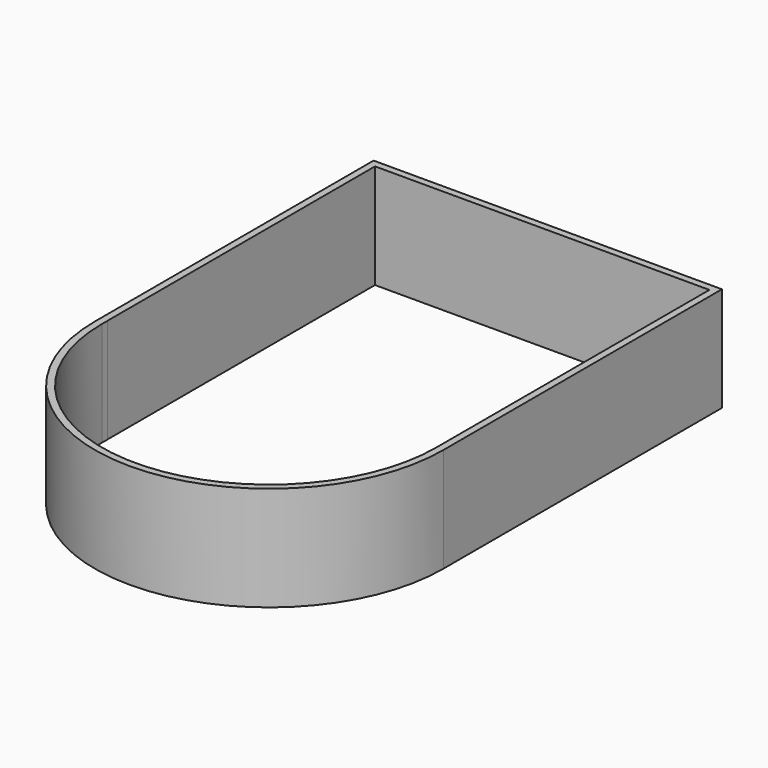
from build123d import *

# Parameters (mm, degrees)
F1_DEPTH = 3000


with BuildPart() as f1:
    # F0 (on Top) → F1 (new body)
    with BuildSketch(Plane.XY):
        with BuildLine():
            Line((5000, 5000), (-5000, 5000))
            Line((-5000, 5000), (-5000, -5000))
            ThreePointArc((-5000, -5000), (-4949.747468, -4292.893219), (-4800, -3600))
            Line((-4800, -3600), (-4800, 4800))
            Line((-4800, 4800), (4800, 4800))
            Line((4800, 4800), (4800, -3600))
            ThreePointArc((4800, -3600), (4949.747468, -4292.893219), (5000, -5000))
            Line((5000, -5000), (5000, 5000))
        make_face()
        with BuildLine():
            ThreePointArc((-4800, -3600), (-4949.747468, -4292.893219), (-5000, -5000))
            Line((-5000, -5000), (-4800, -5000))
            ThreePointArc((-4800, -5000), (-4798.957768, -4899.978282), (-4795.831523, -4800))
            Line((-4795.831523, -4800), (-4800, -4800))
            Line((-4800, -4800), (-4800, -3600))
        make_face()
        with BuildLine():
            Line((4800, -5000), (5000, -5000))
            ThreePointArc((5000, -5000), (4949.747468, -4292.893219), (4800, -3600))
            Line((4800, -3600), (4800, -4800))
            Line((4800, -4800), (4795.831523, -4800))
            ThreePointArc((4795.831523, -4800), (4798.957768, -4899.978282), (4800, -5000))
        make_face()
        with BuildLine():
            Line((-4800, -5000), (-5000, -5000))
            ThreePointArc((-5000, -5000), (0, -10000), (5000, -5000))
            Line((5000, -5000), (4800, -5000))
            ThreePointArc((4800, -5000), (0, -9800), (-4800, -5000))
        make_face()
    extrude(amount=F1_DEPTH)


solid = f1.part
